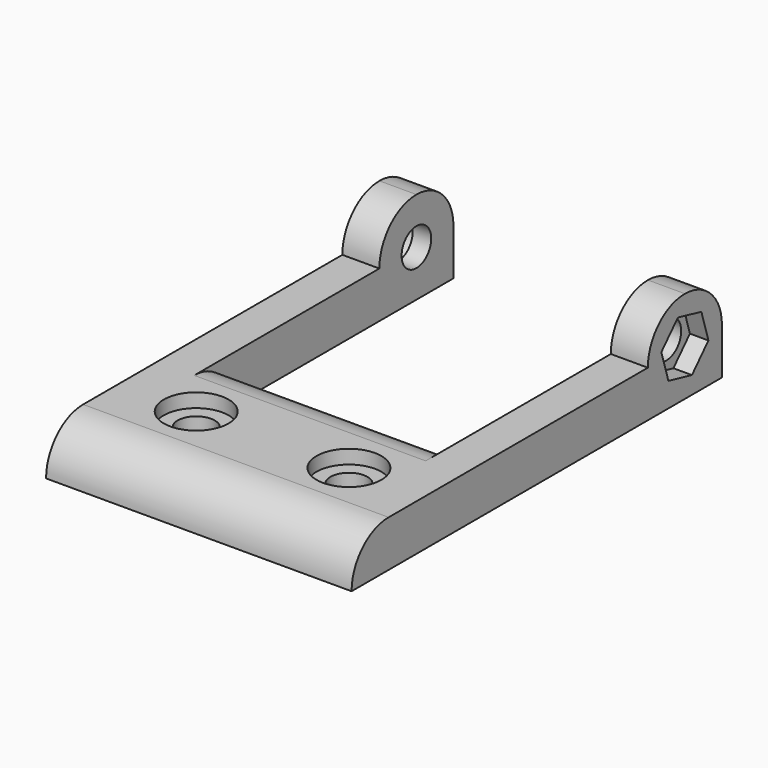
from build123d import *

# Parameters (mm, degrees)
F1_DEPTH        = 5
F2_W            = 10
F2_H            = 10
F3_DEPTH        = 4
F5_D            = 4
F5_CBORE_D      = 6.5
F5_CBORE_DEPTH  = 2
F7_DEPTH        = 4
F9_D            = 4
F10_R           = 2
F11_DEPTH       = 2
F12_R           = 4.99999
F14_D           = 4
F14_CBORE_D     = 7
F14_CBORE_DEPTH = 1.5


# Not quite as in the source:
# - a fillet or chamfer is up to 0.001 mm smaller than in the source, because OpenCascade refuses the exact size


with BuildPart() as f1:
    # F0 (on Top) → F1 (new body)
    with BuildSketch(Plane.XY):
        Polygon((16.5, -25), (16.5, 25), (12.5, 25), (12.5, -5), (-12.5, -5), (-12.5, 25), (-16.5, 25), (-16.5, -25), align=None)
    extrude(amount=F1_DEPTH)

    # F2 (on face) → F3 (join)
    with BuildSketch(Plane(origin=(-16.5, 0, 0), x_dir=(0, -1, 0), z_dir=(-1, 0, 0))):
        with Locations((-20, 5)):
            Rectangle(F2_W, F2_H)
    extrude(amount=-F3_DEPTH)

    # F5 (through all)
    with Locations(Plane(origin=(-16.5, 0, 0), x_dir=(0, -1, 0), z_dir=(-1, 0, 0))):
        with Locations((-20, 5)):
            CounterBoreHole(F5_D / 2, F5_CBORE_D / 2, F5_CBORE_DEPTH)

    # F6 (on face) → F7 (join)
    with BuildSketch(Plane.YZ.offset(16.5)):
        with BuildLine():
            Line((22, 5), (25, 5))
            Line((25, 5), (25, 10))
            Line((25, 10), (15, 10))
            Line((15, 10), (15, 5))
            Line((15, 5), (18, 5))
            ThreePointArc((18, 5), (20, 3), (22, 5))
        make_face()
    extrude(amount=-F7_DEPTH)

    # F9 (through all)
    with Locations(Plane.YZ.offset(16.5)):
        with Locations((20, 5)):
            Hole(F9_D / 2)

    # F10 (on face) → F11 (cut)
    with BuildSketch(Plane.YZ.offset(16.5)):
        Polygon((20.9512871128, 1.8797618421), (23.1778490671, 4.263719727), (22.2265619542, 7.383957885), (19.0487128872, 8.1202381579), (16.8221509329, 5.736280273), (17.7734380458, 2.616042115), align=None)
        with Locations((20, 5)):
            Circle(F10_R, mode=Mode.SUBTRACT)
    extrude(amount=-F11_DEPTH, mode=Mode.SUBTRACT)

    # F12 (radius 5 in the source; OpenCascade refuses exactly that, so slightly less here)
    f12_edges = [f1.edges().sort_by_distance(p)[0] for p in [
        (14.5, 25, 10),
        (14.5, 15, 10),
        (-14.5, 15, 10),
        (-14.5, 25, 10),
        (0, -25, 5),
        (0, -5, 5),
    ]]
    fillet(f12_edges, radius=F12_R)

    # F14 (through all)
    with Locations(Plane.XY.offset(5)):
        with Locations((-8.25, -15.0438509881), (8.25, -15.0438509881)):
            CounterBoreHole(F14_D / 2, F14_CBORE_D / 2, F14_CBORE_DEPTH)


solid = f1.part
